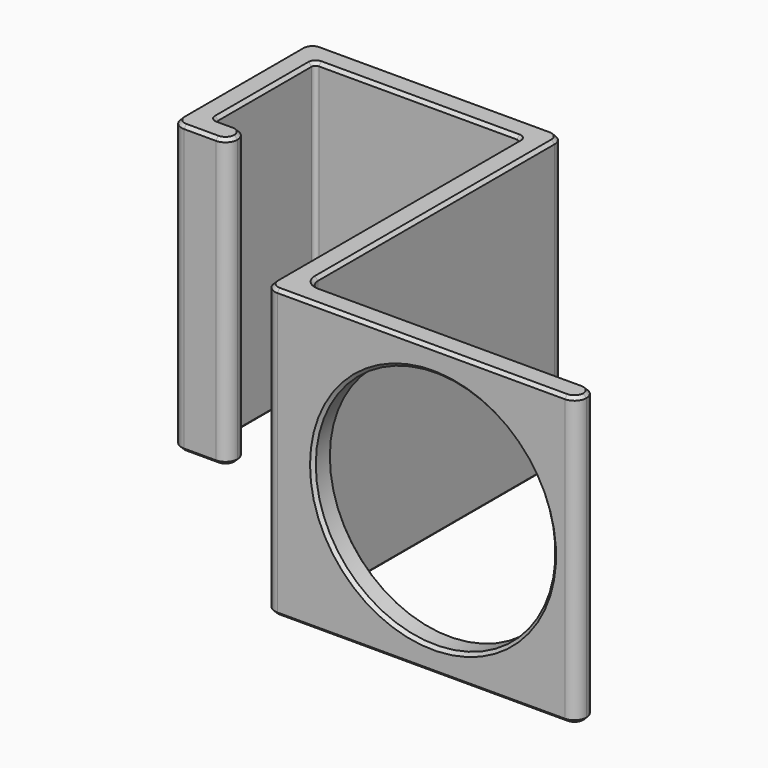
from build123d import *

# Parameters (mm, degrees)
F0_W     = 4
F0_H     = 3
F1_DEPTH = 36
F2_R     = 15
F3_DEPTH = 25
F4_R     = 1.49999
F5_R     = 0.5
F6_SIZE  = 0.4


# Not quite as in the source:
# - a fillet or chamfer is up to 0.001 mm smaller than in the source, because OpenCascade refuses the exact size
# - a feature names something its author has since deleted; it is built from what else it names


with BuildPart() as f1:
    # F0 (on Top) → F1 (new body)
    with BuildSketch(Plane.XY):
        Polygon((-3, 0), (0, 0), (0, 3), (0, 18.6), (25.8, 18.6), (25.8, -21.4), (64.8, -21.4), (64.8, -18.4), (28.8, -18.4), (28.8, 21.6), (-3, 21.6), align=None)
        with Locations((2, 1.5)):
            Rectangle(F0_W, F0_H)
    extrude(amount=F1_DEPTH)

    # F2 (on face) → F3 (cut)
    with BuildSketch(Plane(origin=(0, -18.4, 0), x_dir=(-1, 0, 0), z_dir=(0, 1, 0))):
        with Locations((-46.8, 18)):
            Circle(F2_R)
    extrude(amount=-F3_DEPTH, mode=Mode.SUBTRACT)

    # F4 (radius 1.5 in the source; OpenCascade refuses exactly that, so slightly less here)
    f4_edges = [f1.edges().sort_by_distance(p)[0] for p in [
        (-3, 0, 18),
        (-3, 21.6, 18),
        (28.8, 21.6, 18),
        (28.8, -18.4, 18),
        (25.8, -21.4, 18),
        (4, 3, 18),
        (4, 0, 18),
        (64.8, -21.4, 18),
        (64.8, -18.4, 18),
    ]]
    fillet(f4_edges, radius=F4_R)

    # F5
    f5_edges = [f1.edges().sort_by_distance(p)[0] for p in [
        (0, 18.6, 18),
        (25.8, 18.6, 18),
        (0, 3, 18),
    ]]
    fillet(f5_edges, radius=F5_R)

    # F6
    f6_edges = [f1.edges().sort_by_distance(p)[0] for p in [
        (1.500005, 3, 36),
        (0.146447, 3.146447, 36),
        (3.560663, 2.560663, 36),
        (0, 10.8, 36),
        (4, 1.5, 36),
        (0.146447, 18.453553, 36),
        (3.560663, 0.439337, 36),
        (12.9, 18.6, 36),
        (0.5, 0, 36),
        (25.653553, 18.453553, 36),
        (-2.560663, 0.439337, 36),
        (25.8, -0.900005, 36),
        (-3, 10.8, 36),
        (26.239337, -20.960663, 36),
        (-2.560663, 21.160663, 36),
        (45.3, -21.4, 36),
        (12.9, 21.6, 36),
        (64.360663, -20.960663, 36),
        (28.360663, 21.160663, 36),
        (64.8, -19.9, 36),
        (28.8, 1.6, 36),
        (64.360663, -18.839337, 36),
        (29.239337, -17.960663, 36),
        (46.8, -18.4, 36),
        (1.500005, 3, 0),
        (0.146447, 3.146447, 0),
        (3.560663, 2.560663, 0),
        (0, 10.8, 0),
        (4, 1.5, 0),
        (0.146447, 18.453553, 0),
        (3.560663, 0.439337, 0),
        (12.9, 18.6, 0),
        (0.5, 0, 0),
        (25.653553, 18.453553, 0),
        (-2.560663, 0.439337, 0),
        (25.8, -0.900005, 0),
        (-3, 10.8, 0),
        (26.239337, -20.960663, 0),
        (-2.560663, 21.160663, 0),
        (45.3, -21.4, 0),
        (12.9, 21.6, 0),
        (64.360663, -20.960663, 0),
        (28.360663, 21.160663, 0),
        (64.8, -19.9, 0),
        (28.8, 1.6, 0),
        (64.360663, -18.839337, 0),
        (29.239337, -17.960663, 0),
        (46.8, -18.4, 0),
        (61.8, -18.4, 18),
        (61.8, -21.4, 18),
    ]]
    chamfer(f6_edges, length=F6_SIZE)


solid = f1.part
